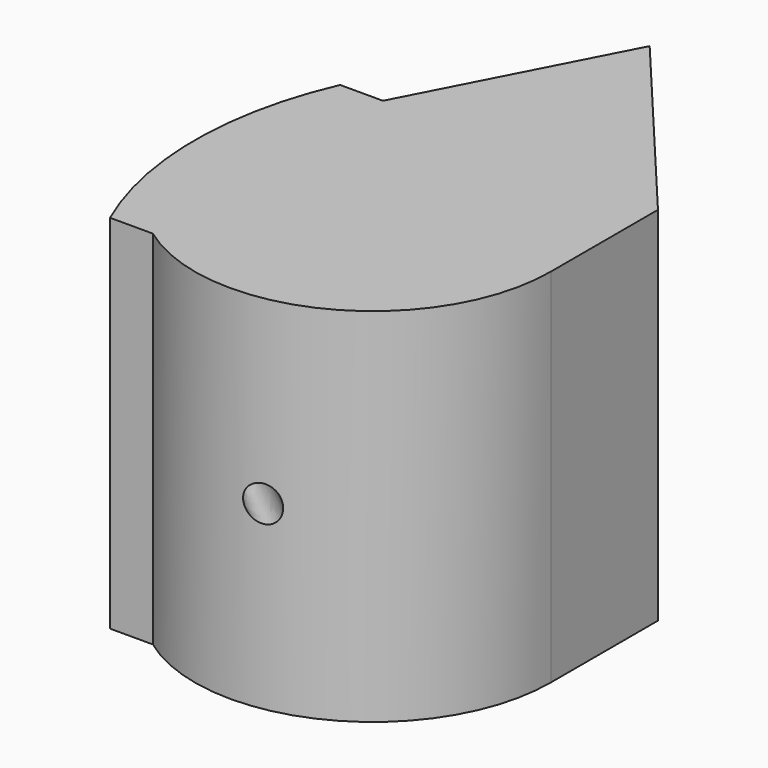
from build123d import *

# Parameters (mm, degrees)
F2_DEPTH      = 25.4
F2_DEPTH_BACK = 25.4
F4_DEPTH      = 50.8
F4_DEPTH_BACK = 50.8
F5_R          = 5
F6_DEPTH      = 127
F7_R          = 31
F8_DEPTH      = 26.5
F9_R          = 5.0038


with BuildPart() as f2:
    # F1 (on Top) → F2 (new body, two sides)
    with BuildSketch(Plane.XY) as f2_sk:
        with BuildLine():
            ThreePointArc((-47.9795897113, -20), (-50, 0), (-47.9795897113, 20))
            Line((-47.9795897113, 20), (-49.9391815056, 20.4))
            ThreePointArc((-49.9391815056, 20.4), (-52, 0), (-49.9391815056, -20.4))
            Line((-49.9391815056, -20.4), (-47.9795897113, -20))
        make_face()
    extrude(amount=F2_DEPTH)
    extrude(f2_sk.sketch, amount=-F2_DEPTH_BACK)


with BuildPart() as f4:
    # F3 (on Top) → F4 (new body, two sides)
    with BuildSketch(Plane.XY) as f4_sk:
        with BuildLine():
            Line((-29.4591242232, 40.4), (-41.4758984651, 40.4))
            ThreePointArc((-41.4758984651, 40.4), (-50, 0), (-41.4758984651, -40.4))
            Line((-41.4758984651, -40.4), (-29.4591242232, -40.4))
            ThreePointArc((-29.4591242232, -40.4), (22.6610214778, -44.569923778), (50, 0))
            Line((50, 0), (50, 37.638230517))
            Line((50, 37.638230517), (0, 97.2259101467))
            Line((0, 97.2259101467), (-29.4591242232, 40.4))
        make_face()
    extrude(amount=F4_DEPTH)
    extrude(f4_sk.sketch, amount=-F4_DEPTH_BACK)

    # F5 (on face) → F6 (cut)
    with BuildSketch(Plane(origin=(47.8744150531, 40.1714040139, 0), x_dir=(-0.6427876097, 0.7660444431, 0), z_dir=(0.7660444431, 0.6427876097, 0))):
        with Locations((32.1393804843, 0)):
            Circle(F5_R)
    extrude(amount=-F6_DEPTH, mode=Mode.SUBTRACT)

    # F7 (on face) → F8 (cut)
    with BuildSketch(Plane(origin=(47.8744150531, 40.1714040139, 0), x_dir=(-0.6427876097, 0.7660444431, 0), z_dir=(0.7660444431, 0.6427876097, 0))):
        with Locations((32.1393804843, 0)):
            Circle(F7_R)
    extrude(amount=-F8_DEPTH, mode=Mode.SUBTRACT)


with BuildPart() as f10_tool:
    # F10: sweep along a path in F0
    with BuildLine(Plane.XY) as f10_path:
        Line((47.5974665938, -81.8939982227), (-50, 0))
    # F9 (on Right) → F10 (sweep)
    with BuildSketch(Plane.YZ):
        with Locations((-41.9549815589, 0)):
            Circle(F9_R)
    sweep(path=f10_path.line)


with BuildPart() as f2_1:
    add(f2.part)

    # F10: cut by f10_tool
    add(f10_tool.part, mode=Mode.SUBTRACT)


with BuildPart() as f4_1:
    add(f4.part)

    # F10: cut by f10_tool
    add(f10_tool.part, mode=Mode.SUBTRACT)


solid = Compound([f2_1.part, f4_1.part])
